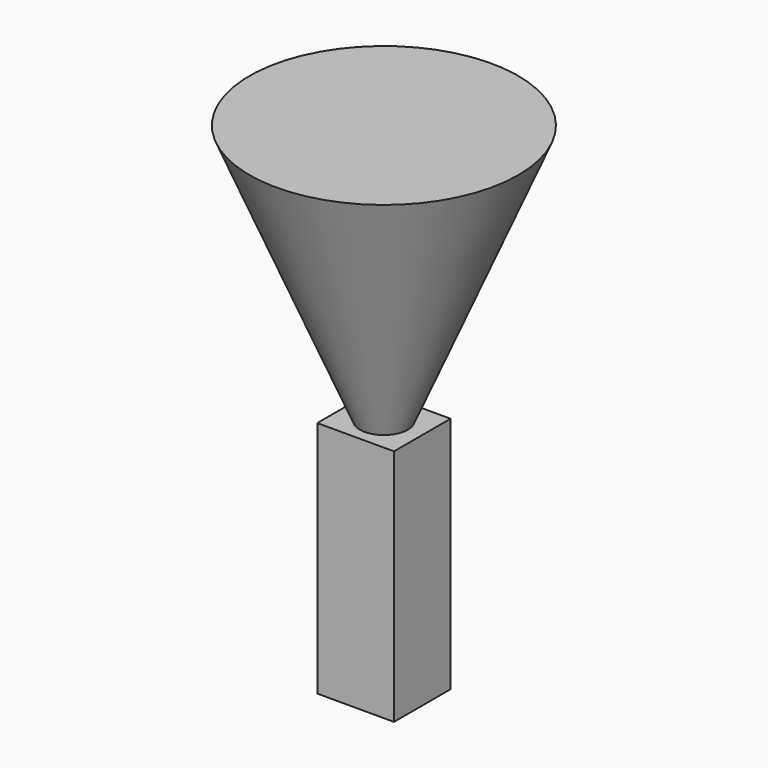
from build123d import *

# Parameters (mm, degrees)
F0_W     = 100.1865565777
F0_H     = 92.3875570297
F1_DEPTH = 311.15
F2_R     = 31.3492715111
F3_DEPTH = 339.6968106
F3_TAPER = -23


# Not quite as in the source:
# - an extrude ends at something that could not be found from the text; its depth is read off the source's solid


with BuildPart() as f1:
    # F0 (on Top) → F1 (new body)
    with BuildSketch(Plane.XY):
        Rectangle(F0_W, F0_H)
    extrude(amount=F1_DEPTH)

    # F2 (on face) → F3 (join, through all)
    with BuildSketch(Plane.XY.offset(311.15)):
        Circle(F2_R)
    extrude(amount=F3_DEPTH, taper=F3_TAPER)


solid = f1.part
